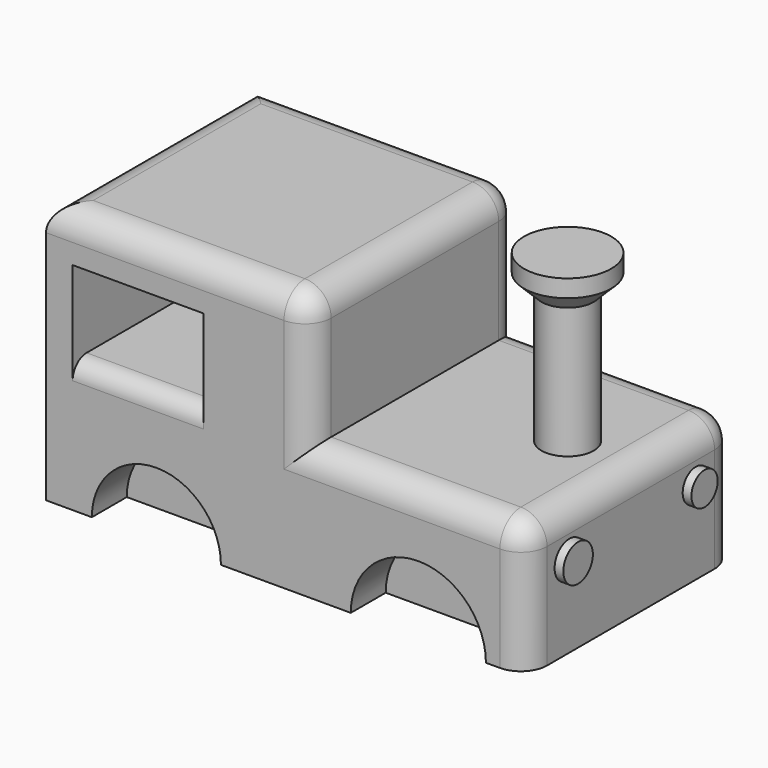
from build123d import *

# Parameters (mm, degrees)
F0_W      = 55
F0_H      = 30
F1_DEPTH  = 30
F2_W      = 24.7374541685
F2_H      = 14.993442893
F3_DEPTH  = 35
F5_DEPTH  = 5
F7_DEPTH  = 5
F8_R      = 3
F9_W      = 15
F9_H      = 9.6639953554
F10_DEPTH = 33.1
F11_R     = 2
F12_R     = 2.1149349852
F12_R_2   = 1.8799425549
F13_DEPTH = 1
F14_R     = 3
F15_DEPTH = 15
F16_R     = 5
F17_DEPTH = 4
F18_SIZE  = 1.99999


# Not quite as in the source:
# - a fillet or chamfer is up to 0.001 mm smaller than in the source, because OpenCascade refuses the exact size


with BuildPart() as f1:
    # F0 (on Top) → F1 (new body)
    with BuildSketch(Plane.XY):
        with Locations((5.7581346482, 7.7498872403)):
            Rectangle(F0_W, F0_H)
    extrude(amount=F1_DEPTH)

    # F2 (on face) → F3 (cut)
    with BuildSketch(Plane(origin=(0, 22.7498872403, 0), x_dir=(-1, 0, 0), z_dir=(0, 1, 0))):
        with Locations((-20.889407564, 22.5032785535)):
            Rectangle(F2_W, F2_H)
    extrude(amount=-F3_DEPTH, mode=Mode.SUBTRACT)

    # F4 (on face) → F5 (cut)
    with BuildSketch(Plane(origin=(0, 22.7498872403, 0), x_dir=(-1, 0, 0), z_dir=(0, 1, 0))):
        with BuildLine():
            Line((-27.9546213446, 0), (-12.7694251838, 0))
            ThreePointArc((-12.7694251838, 0), (-20.3620232642, 7.5925980804), (-27.9546213446, 0))
        make_face()
        with BuildLine():
            ThreePointArc((17.3747475732, 0), (9.9283689633, 7.4463786099), (2.4819903534, 0))
            Line((2.4819903534, 0), (17.3747475732, 0))
        make_face()
    extrude(amount=-F5_DEPTH, mode=Mode.SUBTRACT)

    # F6 (on face) → F7 (cut)
    with BuildSketch(Plane.XZ.offset(7.2501127597)):
        with BuildLine():
            Line((-16.4975558603, 0), (-1.7069804287, 0))
            ThreePointArc((-1.7069804287, 0), (-9.1022681445, 7.3952877158), (-16.4975558603, 0))
        make_face()
        with BuildLine():
            ThreePointArc((28.6537096156, 0), (20.9127571434, 7.7409524722), (13.1718046712, 0))
            Line((13.1718046712, 0), (28.6537096156, 0))
        make_face()
    extrude(amount=-F7_DEPTH, mode=Mode.SUBTRACT)

    # F8
    f8_edges = [f1.edges().sort_by_distance(p)[0] for p in [
        (8.52068, -7.250113, 22.503279),
        (8.52068, 22.749887, 22.503279),
        (33.258135, 22.749887, 7.503279),
        (33.258135, 7.749887, 15.006557),
        (33.258135, -7.250113, 7.503279),
        (8.52068, 7.749887, 30),
        (-6.610592, 22.749887, 30),
        (-21.741865, 7.749887, 30),
        (20.889408, 22.749887, 15.006557),
        (20.889408, -7.250113, 15.006557),
        (-6.610592, -7.250113, 30),
    ]]
    fillet(f8_edges, radius=F8_R)

    # F9 (on face) → F10 (cut)
    with BuildSketch(Plane.XZ.offset(7.2501127597)):
        with Locations((-11.2023635954, 19.8851507157)):
            Rectangle(F9_W, F9_H)
    extrude(amount=-F10_DEPTH, mode=Mode.SUBTRACT)

    # F11
    f11_edges = [f1.edges().sort_by_distance(p)[0] for p in [
        (-11.202364, 22.749887, 15.053153),
        (-11.202364, -7.250113, 15.053153),
    ]]
    fillet(f11_edges, radius=F11_R)

    # F12 (on face) → F13 (join)
    with BuildSketch(Plane.YZ.offset(33.2581346482)):
        with Locations((-1.053063781, 9.3823140487)):
            Circle(F12_R)
        with Locations((17.056318, 9.5132254064)):
            Circle(F12_R_2)
    extrude(amount=F13_DEPTH)

    # F14 (on face) → F15 (join)
    with BuildSketch(Plane.XY.offset(15.006557107)):
        with Locations((25.5206804797, 8.3661237732)):
            Circle(F14_R)
    extrude(amount=F15_DEPTH)

    # F16 (on face) → F17 (join)
    with BuildSketch(Plane.XY.offset(30.006557107)):
        with Locations((25.5206804797, 8.3661237732)):
            Circle(F16_R)
    extrude(amount=F17_DEPTH)

    # F18 (size 2 in the source; OpenCascade refuses exactly that, so slightly less here)
    f18_edges = [f1.edges().sort_by_distance(p)[0] for p in [
        (20.52068, 8.366124, 30.006557),
    ]]
    chamfer(f18_edges, length=F18_SIZE)


solid = f1.part
